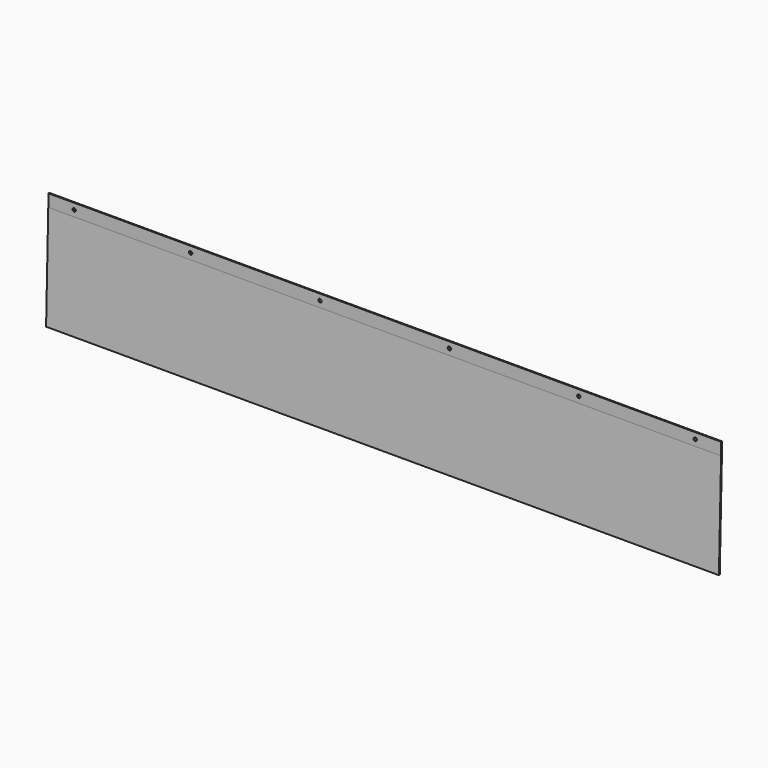
from build123d import *

# Parameters (mm, degrees)
F1_DEPTH    = 650
F2_R        = 3.25
F3_DEPTH    = 25
F4_T1_DEPTH = 1300
F5_T1_DEPTH = 1300.2618143417


# Not quite as in the source:
# - a fillet or chamfer that OpenCascade refuses, or shapes differently, is made with other operations: its cross-section is extruded or revolved along the edge and cut away or added


with BuildPart() as f1:
    # F0 (on Right) → F1 (new body, symmetric)
    with BuildSketch(Plane.YZ):
        Polygon((0, -24), (0, 0), (-2, 0), (-2, -23.9738185658), (-7.2608812598, -224.8787684235), (-5.2615666099, -224.9311223201), align=None)
    extrude(amount=F1_DEPTH, both=True)

    # F2 (on face) → F3 (cut)
    with BuildSketch(Plane(origin=(0, 0, 0), x_dir=(-1, 0, 0), z_dir=(0, 1, 0))):
        with Locations((-600, -12)):
            Circle(F2_R)
        with Locations((-375, -12)):
            Circle(F2_R)
        with Locations((-125, -12)):
            Circle(F2_R)
        with Locations((600, -12)):
            Circle(F2_R)
        with Locations((375, -12)):
            Circle(F2_R)
        with Locations((125, -12)):
            Circle(F2_R)
    extrude(amount=-F3_DEPTH, mode=Mode.SUBTRACT)

    # F4: fillet of radius 2 on 1 edges, made by hand

    # F4_s2 → F4_t1 (join)
    with BuildSketch(Plane.YZ.offset(-650)):
        with BuildLine():
            ThreePointArc((-2, -23.9476371317), (-2.0001713449, -23.9738163228), (-2.00068535, -23.9999910283))
            Line((-2.00068535, -23.9999910283), (-2, -23.9738185658))
            Line((-2, -23.9738185658), (-2, -23.9476371317))
        make_face()
    extrude(amount=F4_T1_DEPTH)

    # F5: fillet of radius 4 on 1 edges, made by hand

    # F5_s2 → F5_t1 (cut)
    with BuildSketch(Plane.YZ.offset(-650.1309071708)):
        with BuildLine():
            ThreePointArc((-0.0013707001, -24.0523449249), (-0.0003426897, -23.9999955139), (0, -23.9476371317))
            Line((0, -23.9476371317), (0, -24))
            Line((0, -24), (-0.0013707001, -24.0523449249))
        make_face()
    extrude(amount=F5_T1_DEPTH, mode=Mode.SUBTRACT)


solid = f1.part
